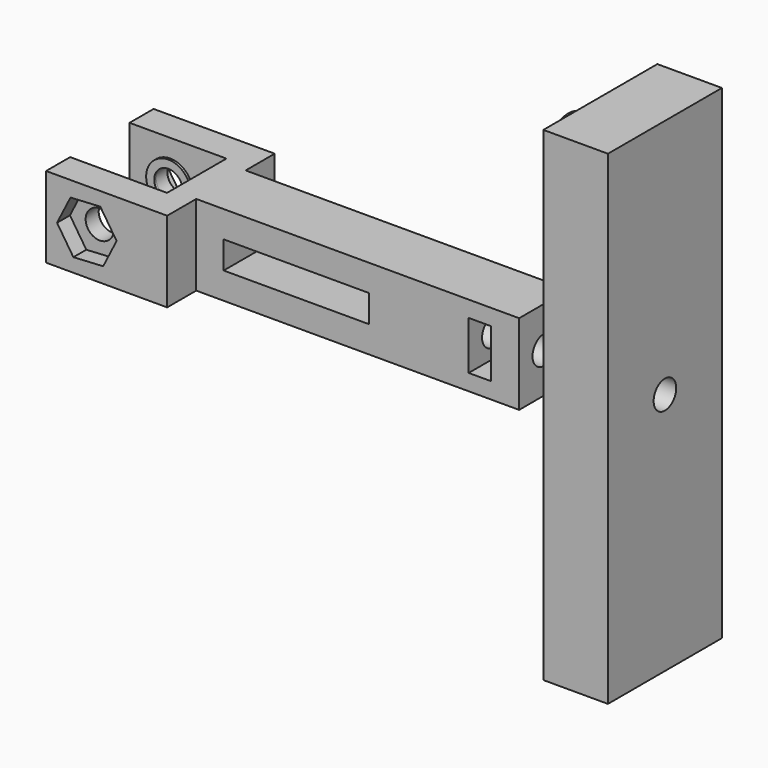
from build123d import *

# Parameters (mm, degrees)
F0_W      = 40
F0_H      = 3.825
F1_DEPTH  = 10
F2_R      = 1.75
F3_DEPTH  = 16.651
F4_W      = 18
F4_H      = 3.4
F4_W_2    = 2.75
F4_H_2    = 6
F5_DEPTH  = 12.151
F6_R      = 1.75
F7_DEPTH  = 15
F10_DEPTH = 2
F11_W     = 17.65
F11_H     = 60
F12_DEPTH = 8
F13_R     = 1.75
F14_DEPTH = 70.001
F15_R     = 2.75
F15_R_2   = 1.75
F16_DEPTH = 0.3
F17_R     = 1.75
F18_DEPTH = 2
F19_R     = 3.75
F20_DEPTH = 4


# Not quite as in the source:
# - a pattern or mirror of a feature is missing from the dataset's text; its kind, count and spacing are read off the source's solid


with BuildPart() as f1:
    # F0 (on Top) → F1 (new body)
    with BuildSketch(Plane.XY):
        Polygon((0, -3.825), (0, 0), (-3, 0), (-3, -4.6), (-15, -4.6), (-15, -8.325), (0, -8.325), align=None)
        Polygon((-3, 0), (0, 0), (0, 3.825), (0, 8.325), (-15, 8.325), (-15, 4.6), (-3, 4.6), align=None)
        with Locations((20, 1.9125)):
            Rectangle(F0_W, F0_H)
        with Locations((20, -1.9125)):
            Rectangle(F0_W, F0_H)
    extrude(amount=F1_DEPTH)

    # F2 (on face) → F3 (cut, through all)
    with BuildSketch(Plane.XZ.offset(8.325)):
        with Locations((-9.9527407438, 5)):
            Circle(F2_R)
    extrude(amount=-F3_DEPTH, mode=Mode.SUBTRACT)

    # F4 (on face) → F5 (cut, through all)
    with BuildSketch(Plane.XZ.offset(3.825)):
        with Locations((12.4002694301, 5)):
            Rectangle(F4_W, F4_H)
        with Locations((35.125, 5)):
            Rectangle(F4_W_2, F4_H_2)
    extrude(amount=-F5_DEPTH, mode=Mode.SUBTRACT)

    # F6 (on face) → F7 (cut)
    with BuildSketch(Plane.YZ.offset(40)):
        with Locations((0, 5)):
            Circle(F6_R)
    extrude(amount=-F7_DEPTH, mode=Mode.SUBTRACT)

    # F15 (on face) → F16 (join)
    with BuildSketch(Plane.XZ.offset(-4.6)):
        with Locations((-9.9527407438, 5)):
            Circle(F15_R)
        with Locations((-9.9527407438, 5)):
            Circle(F15_R_2, mode=Mode.SUBTRACT)
    f16 = extrude(amount=F16_DEPTH)

    # F16_copies: F16 across plane
    add(f16.mirror(Plane(origin=(0, 0, 0), x_dir=(0, 0, -1), z_dir=(0, -1, 0))))

    # F17 (on face) → F18 (cut)
    with BuildSketch(Plane.XZ.offset(8.325)):
        Polygon((-7.9284293953, 1.9088033227), (-6.2635302189, 5.2075067143), (-8.2878415673, 8.2987033916), (-11.9770520922, 8.0911966773), (-13.6419512686, 4.7924932857), (-11.6176399202, 1.7012966084), align=None)
        with Locations((-9.9527407438, 5)):
            Circle(F17_R, mode=Mode.SUBTRACT)
    f18 = extrude(amount=-F18_DEPTH, mode=Mode.SUBTRACT)

    # F18_copies: F18 across plane
    add(f18.mirror(Plane.ZX), mode=Mode.SUBTRACT)


with BuildPart() as f10:
    # F9 (on offset) → F10 (new body)
    with BuildSketch(Plane.YZ.offset(45)):
        Polygon((3.825, 0), (3.825, 10), (3.825, 19.8484882712), (-3.825, 19.8484882712), (-3.825, 10), (-3.825, 0), (-3.825, -10.1515117288), (3.825, -10.1515117288), align=None)
    extrude(amount=F10_DEPTH)

    # F11 (on face) → F12 (join)
    with BuildSketch(Plane.YZ.offset(47)):
        with Locations((0, 4.8484882712)):
            Rectangle(F11_W, F11_H)
    extrude(amount=F12_DEPTH)

    # F13 (on face) → F14 (cut, through all)
    with BuildSketch(Plane.YZ.offset(55)):
        with Locations((0, 5)):
            Circle(F13_R)
    extrude(amount=-F14_DEPTH, mode=Mode.SUBTRACT)

    # F19 (on face) → F20 (join)
    with BuildSketch(Plane(origin=(47, 0, 0), x_dir=(0, -1, 0), z_dir=(-1, 0, 0))):
        with Locations((0, 28)):
            Circle(F19_R)
        with Locations((0, -18)):
            Circle(F19_R)
    extrude(amount=F20_DEPTH)


solid = Compound([f1.part, f10.part])
